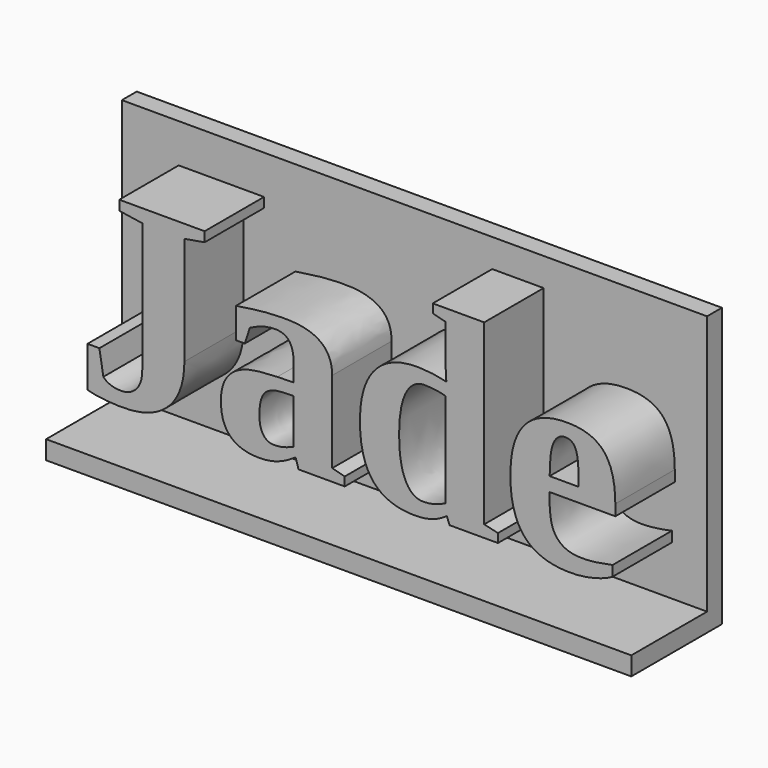
from build123d import *

# Parameters (mm, degrees)
F0_TEXT_SIZE = 73.653521559
F1_DEPTH     = 25
F2_W         = 157.5665358781
F2_H         = 70
F3_DEPTH     = 5
F4_W         = 157.56654
F4_H         = 5
F5_DEPTH     = 30.5


# Not quite as in the source:
# - Text() gives the source's letters only with a copy of the font that has no kerning and outlines rounded to 1/6400 em; it was checked with that copy


with BuildPart() as f1:
    # F0 (on Front) → F1 (new body)
    with BuildSketch(Plane.XZ):
        with Locations((-59.0219639134, -14.6598838275)):
            Text('Jade', F0_TEXT_SIZE, font='Tinos', font_style=FontStyle.BOLD, text_align=(TextAlign.LEFT, TextAlign.BOTTOM))
    extrude(amount=F1_DEPTH)

    # F2 (on Front) → F3 (join)
    with BuildSketch(Plane.XZ):
        with Locations((16.2882208824, 9.0647488832)):
            Rectangle(F2_W, F2_H)
    extrude(amount=F3_DEPTH)

    # F4 (on face) → F5 (join)
    with BuildSketch(Plane(origin=(0, 0, 0), x_dir=(-1, 0, 0), z_dir=(0, 1, 0))):
        with Locations((-16.2882188214, -28.4352511168)):
            Rectangle(F4_W, F4_H)
    extrude(amount=-F5_DEPTH)


solid = f1.part
